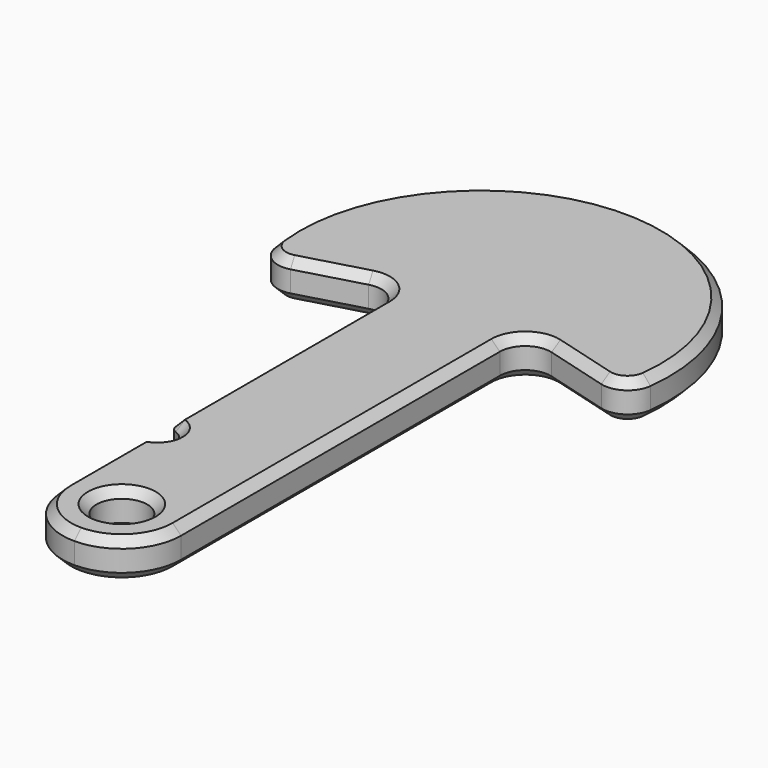
from build123d import *

# Parameters (mm, degrees)
F0_R     = 1.5
F1_DEPTH = 2.25
F2_R     = 1.5
F3_SIZE  = 0.49999


# Not quite as in the source:
# - a fillet or chamfer is up to 0.001 mm smaller than in the source, because OpenCascade refuses the exact size


with BuildPart() as f1:
    # F0 (on Top) → F1 (new body)
    with BuildSketch(Plane.XY):
        with BuildLine():
            Line((3.5, -0.9777600189), (10.7388314076, -3))
            ThreePointArc((10.7388314076, -3), (0, 11.15), (-10.7388314076, -3))
            Line((-10.7388314076, -3), (-3.5, -0.9777600189))
            Line((-3.5, -0.9777600189), (-3.5, -18.0857864376))
            ThreePointArc((-3.5, -18.0857864376), (-3.4082482905, -18.3744615722), (-3.1666666667, -18.5571909584))
            ThreePointArc((-3.1666666667, -18.5571909584), (-2.5, -19.5), (-3.1666666667, -20.4428090416))
            ThreePointArc((-3.1666666667, -20.4428090416), (-3.4082482905, -20.6255384278), (-3.5, -20.9142135624))
            Line((-3.5, -20.9142135624), (-3.5, -26.5))
            ThreePointArc((-3.5, -26.5), (-2.4748737342, -28.9748737342), (0, -30))
            ThreePointArc((0, -30), (2.4748737342, -28.9748737342), (3.5, -26.5))
            Line((3.5, -26.5), (3.5, -0.9777600189))
        make_face()
        with Locations((0, -26.5)):
            Circle(F0_R, mode=Mode.SUBTRACT)
    extrude(amount=F1_DEPTH)

    # F2
    f2_edges = [f1.edges().sort_by_distance(p)[0] for p in [
        (10.738831, -3, 1.125),
        (-10.738831, -3, 1.125),
        (-3.5, -0.97776, 1.125),
        (3.5, -0.97776, 1.125),
    ]]
    fillet(f2_edges, radius=F2_R)

    # F3 (size 0.5 in the source; OpenCascade refuses exactly that, so slightly less here)
    f3_edges = [f1.edges().sort_by_distance(p)[0] for p in [
        (3.5, -14.727116, 2.25),
        (4.093187, -1.759372, 2.25),
        (0, -30, 2.25),
        (7.292383, -2.0372, 2.25),
        (-3.5, -23.707107, 2.25),
        (10.420577, -2.365727, 2.25),
        (-3.408248, -20.625538, 2.25),
        (0, 11.15, 2.25),
        (-2.5, -19.5, 2.25),
        (-10.420577, -2.365727, 2.25),
        (-3.408248, -18.374462, 2.25),
        (-7.292383, -2.0372, 2.25),
        (-3.5, -10.520009, 2.25),
        (-4.093187, -1.759372, 2.25),
        (-1.5, -26.5, 2.25),
        (3.5, -14.727116, 0),
        (4.093187, -1.759372, 0),
        (0, -30, 0),
        (7.292383, -2.0372, 0),
        (-3.5, -23.707107, 0),
        (10.420577, -2.365727, 0),
        (-3.408248, -20.625538, 0),
        (0, 11.15, 0),
        (-2.5, -19.5, 0),
        (-10.420577, -2.365727, 0),
        (-3.408248, -18.374462, 0),
        (-7.292383, -2.0372, 0),
        (-3.5, -10.520009, 0),
        (-4.093187, -1.759372, 0),
        (-1.5, -26.5, 0),
    ]]
    chamfer(f3_edges, length=F3_SIZE)


solid = f1.part
